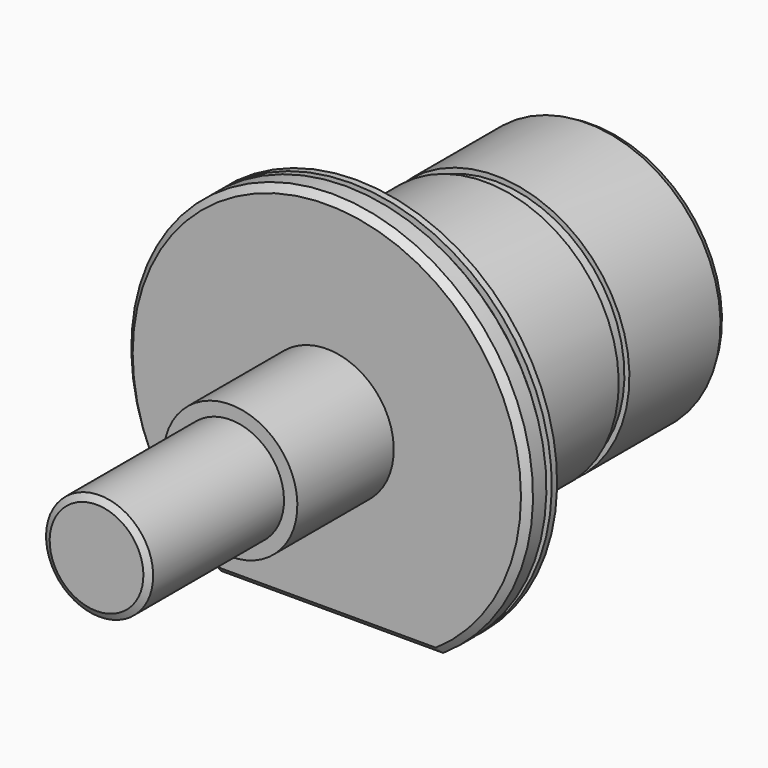
from build123d import *

# Parameters (mm, degrees)
F2_W        = 60
F2_H        = 10
F3_DEPTH    = 92.501
F4_SIZE     = 1
F5_C1_SIZE2 = 1
F5_C1_SIZE  = 0.5773502692
F5_C2_SIZE2 = 0.5773502692
F5_C2_SIZE  = 1
F6_W        = 2
F6_H        = 2
F8_R        = 20.3
F9_DEPTH    = 1


with BuildPart() as f1:
    # F0 (on Right) → F1 (revolve)
    with BuildSketch(Plane.YZ):
        Polygon((92.5, 0), (0, 0), (0, -8), (25, -8), (25, -10), (43, -10), (43, -30), (47.5, -30), (47.5, -20), (92.5, -20), align=None)
    revolve(axis=Axis((0, 37.7989597619, 0), (0, 1, 0)))

    # F2 (on Front) → F3 (cut, through all)
    with BuildSketch(Plane.XZ):
        with Locations((0, -30)):
            Rectangle(F2_W, F2_H)
    extrude(amount=-F3_DEPTH, mode=Mode.SUBTRACT)

    # F4
    f4_edges = [f1.edges().sort_by_distance(p)[0] for p in [
        (0, 47.5, 30),
        (0, 47.5, -25),
        (0, 43, 30),
        (0, 43, -25),
    ]]
    chamfer(f4_edges, length=F4_SIZE)

    # F5: chamfer of 1 x 0.5773502692 on 2 edges, made by hand

    # F5_c1
    f5_c1_edges = [f1.edges().sort_by_distance(p)[0] for p in [
        (0, 0, 8),
    ]]
    f5_c1_side = f1.faces().sort_by_distance((0, 0.0115470054, 8))[0]
    chamfer(f5_c1_edges, length=F5_C1_SIZE, length2=F5_C1_SIZE2, reference=f5_c1_side)

    # F5_c2
    f5_c2_edges = [f1.edges().sort_by_distance(p)[0] for p in [
        (0, 92.5, 20),
    ]]
    f5_c2_side = f1.faces().sort_by_distance((0, 92.4884529946, 20))[0]
    chamfer(f5_c2_edges, length=F5_C2_SIZE, length2=F5_C2_SIZE2, reference=f5_c2_side)

    # F6 (on Right) → F7 (revolve, cut)
    with BuildSketch(Plane.YZ):
        with Locations((73.5, 20.25)):
            Rectangle(F6_W, F6_H)
    revolve(axis=Axis((0, 66.5382612497, 0), (0, -1, 0)), mode=Mode.SUBTRACT)


with BuildPart() as f9:
    # F8 (on face) → F9 (new body)
    with BuildSketch(Plane(origin=(0, 47.5, 0), x_dir=(-1, 0, 0), z_dir=(0, 1, 0))):
        with BuildLine():
            ThreePointArc((16.5831239518, -25), (0, 30), (-16.5831239518, -25))
            Line((-16.5831239518, -25), (16.5831239518, -25))
        make_face()
        Circle(F8_R, mode=Mode.SUBTRACT)
    extrude(amount=F9_DEPTH)


solid = Compound([f1.part, f9.part])
